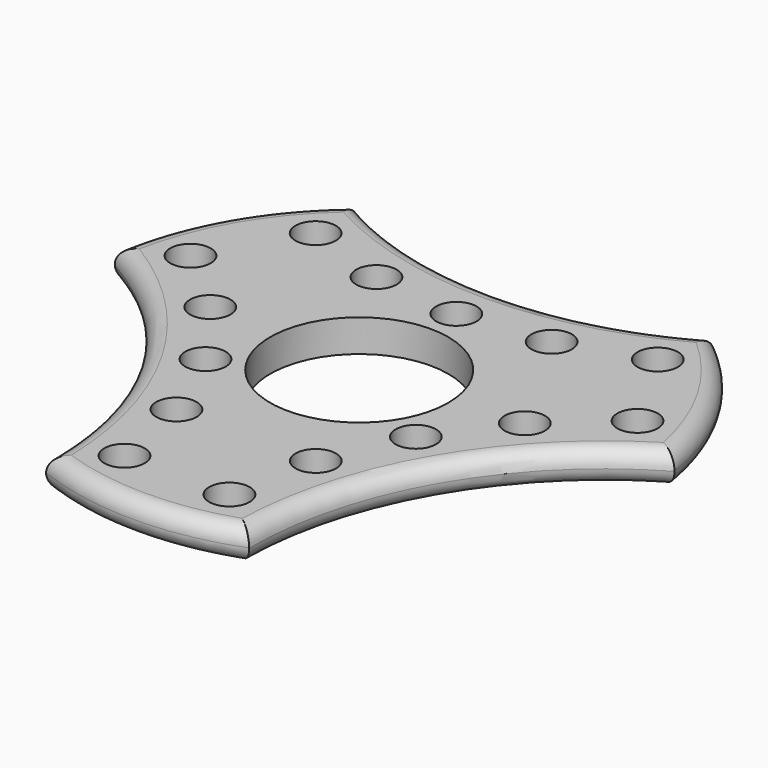
from build123d import *

# Parameters (mm, degrees)
F0_R     = 2.5
F0_R_2   = 11
F1_DEPTH = 2
F2_R     = 1.99999


# Not quite as in the source:
# - a fillet or chamfer is up to 0.001 mm smaller than in the source, because OpenCascade refuses the exact size


with BuildPart() as f1:
    # F0 (on Top) → F1 (new body, symmetric)
    with BuildSketch(Plane.XY):
        with BuildLine():
            ThreePointArc((22.0269415402, 27.1995192308), (0, 21.25), (-22.0269415402, 27.1995192308))
            ThreePointArc((-22.0269415402, 27.1995192308), (-30.3108891325, 17.5), (-34.5689453947, 5.4761313261))
            ThreePointArc((-34.5689453947, 5.4761313261), (-18.4030398304, -10.625), (-12.5420038545, -32.6756505569))
            ThreePointArc((-12.5420038545, -32.6756505569), (0, -35), (12.5420038545, -32.6756505569))
            ThreePointArc((12.5420038545, -32.6756505569), (18.4030398304, -10.625), (34.5689453947, 5.4761313261))
            ThreePointArc((34.5689453947, 5.4761313261), (30.3108891325, 17.5), (22.0269415402, 27.1995192308))
        make_face()
        with Locations((-6.4819163414, -28.1422128626)):
            Circle(F0_R, mode=Mode.SUBTRACT)
        with Locations((-8.6058037086, -17.4647100248)):
            Circle(F0_R, mode=Mode.SUBTRACT)
        with Locations((-12.9903810568, -7.5)):
            Circle(F0_R, mode=Mode.SUBTRACT)
        with Locations((6.4819163414, -28.1422128626)):
            Circle(F0_R, mode=Mode.SUBTRACT)
        with Locations((8.6058037086, -17.4647100248)):
            Circle(F0_R, mode=Mode.SUBTRACT)
        with Locations((12.9903810568, -7.5)):
            Circle(F0_R, mode=Mode.SUBTRACT)
        with Locations((-19.4277844055, 1.2795103808)):
            Circle(F0_R, mode=Mode.SUBTRACT)
        with Locations((-27.6128294284, 8.4576022144)):
            Circle(F0_R, mode=Mode.SUBTRACT)
        with Locations((-21.130913087, 19.6846106482)):
            Circle(F0_R, mode=Mode.SUBTRACT)
        with Locations((-10.8219806969, 16.185199644)):
            Circle(F0_R, mode=Mode.SUBTRACT)
        Circle(F0_R_2, mode=Mode.SUBTRACT)
        with Locations((19.4277844055, 1.2795103808)):
            Circle(F0_R, mode=Mode.SUBTRACT)
        with Locations((27.6128294284, 8.4576022144)):
            Circle(F0_R, mode=Mode.SUBTRACT)
        with Locations((0, 15)):
            Circle(F0_R, mode=Mode.SUBTRACT)
        with Locations((10.8219806969, 16.185199644)):
            Circle(F0_R, mode=Mode.SUBTRACT)
        with Locations((21.130913087, 19.6846106482)):
            Circle(F0_R, mode=Mode.SUBTRACT)
    extrude(amount=F1_DEPTH, both=True)

    # F2 (radius 2 in the source; OpenCascade refuses exactly that, so slightly less here)
    f2_edges = [f1.edges().sort_by_distance(p)[0] for p in [
        (0, -35, 2),
        (-18.40304, -10.625, 2),
        (30.310889, 17.5, 2),
        (-18.40304, -10.625, -2),
        (0, 21.25, -2),
        (0, 21.25, 2),
        (-30.310889, 17.5, -2),
        (-30.310889, 17.5, 2),
        (30.310889, 17.5, -2),
        (18.40304, -10.625, 2),
        (18.40304, -10.625, -2),
        (0, -35, -2),
    ]]
    fillet(f2_edges, radius=F2_R)


solid = f1.part
